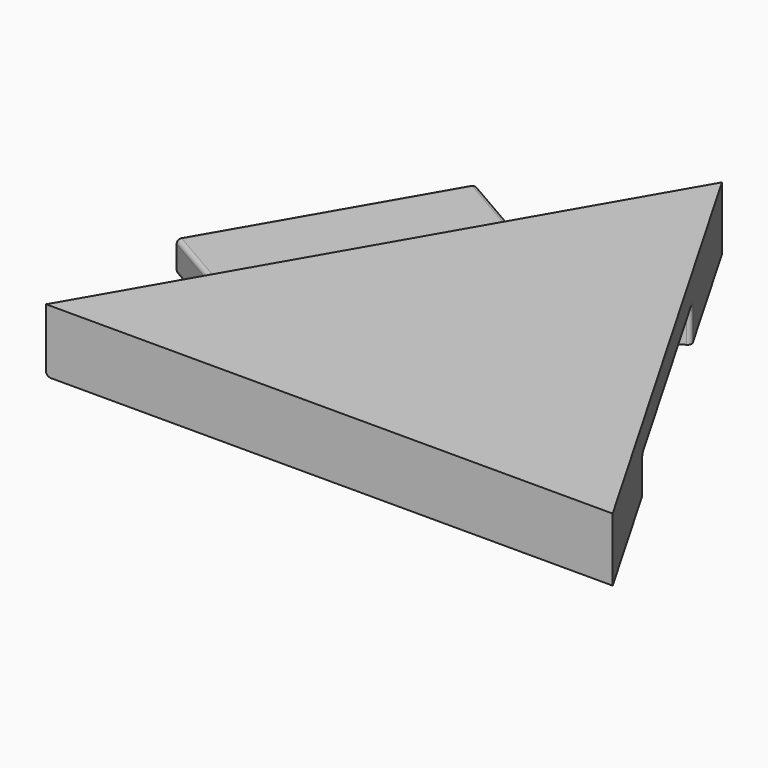
from build123d import *

# Parameters (mm, degrees)
F1_DEPTH = 19.2024
F2_W     = 77.47
F2_H     = 10.16
F3_DEPTH = 39.37
F4_F1_R  = 1.27
F4_F2_R  = 1.27
F5_W     = 76.2
F5_H     = 9.525
F6_DEPTH = 38.1
F7_R     = 1.27


with BuildPart() as f1:
    # F0 (on Top) → F1 (new body)
    with BuildSketch(Plane.XY):
        Polygon((-85.725, -49.4933518263), (85.725, -49.4933518263), (0, 98.9867036526), align=None)
    extrude(amount=F1_DEPTH)

    # F2 (on face) → F3 (cut)
    with BuildSketch(Plane(origin=(42.8625, 24.7466759131, 0), x_dir=(-0.5, 0.8660254038, 0), z_dir=(0.8660254038, 0.5, 0))):
        with Locations((0, 5.08)):
            Rectangle(F2_W, F2_H)
    extrude(amount=-F3_DEPTH, mode=Mode.SUBTRACT)

    # F4: fillet of radius 1.27 on 6 edges, made by hand

    # F4_f1
    f4_f1_edges = [f1.edges().sort_by_distance(p)[0] for p in [
        (45.1822899265, -18.6413181024, 10.16),
        (28.134579853, -28.4838181024, 5.08),
        (8.767079853, 5.0616759131, 10.16),
        (6.4472899265, 48.4496699287, 10.16),
        (-10.600420147, 38.6071699287, 5.08),
    ]]
    fillet(f4_f1_edges, radius=F4_F1_R)

    # F4_f2
    f4_f2_edges = [f1.edges().sort_by_distance(p)[0] for p in [
        (62.23, -8.7988181024, 4.445),
        (62.0440128061, -8.476678833, 9.7880256121),
    ]]
    fillet(f4_f2_edges, radius=F4_F2_R)

    # F5 (on face) → F6 (join)
    with BuildSketch(Plane(origin=(-42.8625, 24.7466759131, 0), x_dir=(-0.5, -0.8660254038, 0), z_dir=(-0.8660254038, 0.5, 0))):
        with Locations((0, 4.7625)):
            Rectangle(F5_W, F5_H)
    extrude(amount=F6_DEPTH)

    # F7
    f7_edges = [f1.edges().sort_by_distance(p)[0] for p in [
        (-75.858068, 43.796676, 9.525),
        (-56.808068, 76.792244, 4.7625),
        (-75.858068, 43.796676, 0),
        (-94.908068, 10.801108, 4.7625),
        (-40.310284, 67.267244, 9.525),
        (-78.410284, 1.276108, 0),
        (-23.8125, 57.742244, 4.7625),
        (-61.9125, -8.248892, 4.7625),
        (-78.410284, 1.276108, 9.525),
        (-73.81875, -28.871122, 0),
        (-42.8625, 24.746676, 9.525),
    ]]
    fillet(f7_edges, radius=F7_R)


solid = f1.part
